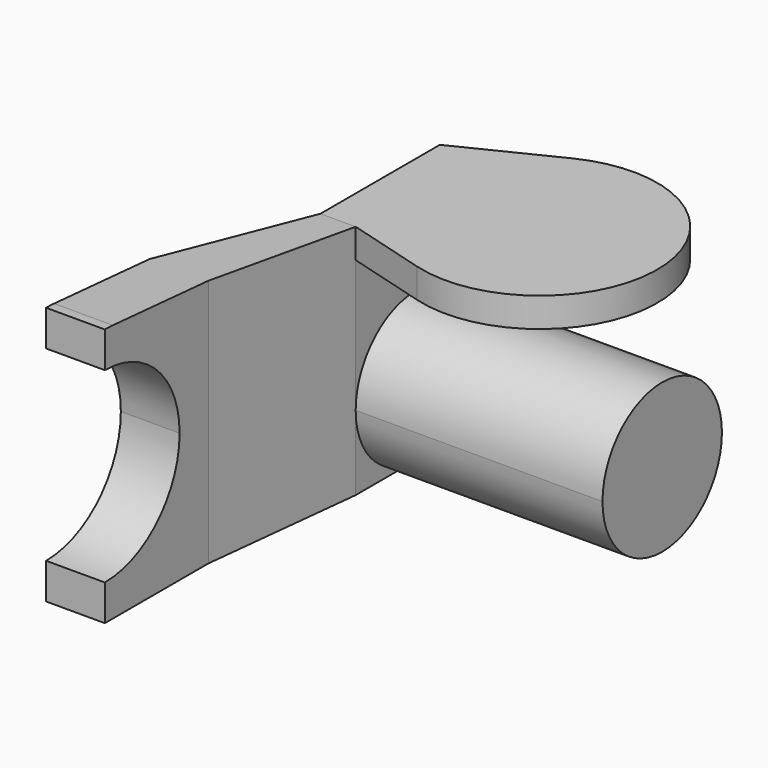
from build123d import *

# Parameters (mm, degrees)
F1_DEPTH      = 10
F2_DEPTH      = 3
F2_DEPTH_BACK = 3
F1_FACE_W     = 10
F1_FACE_H     = 42.3516603272
F2_FACE_W     = 6
F2_FACE_H     = 40.2
F5_DEPTH      = 5
F6_START      = 2
F6_DEPTH      = 43
F8_DEPTH      = 5


# Not quite as in the source:
# - a feature names something its author has since deleted; it is built from what else it names


with BuildPart() as f1:
    # F0 (on Right) → F1 (new body)
    with BuildSketch(Plane.YZ):
        with BuildLine():
            ThreePointArc((15.9, 0), (11.2429978209, -11.2429978209), (0, -15.9))
            Line((0, -15.9), (0, -22))
            ThreePointArc((0, -22), (15.5563491861, -15.5563491861), (22, 0))
            ThreePointArc((22, 0), (16.1495801051, 14.9395803966), (1.7099034157, 21.9334500321))
            ThreePointArc((1.7099034157, 21.9334500321), (0.8555989991, 21.9833562122), (0, 22))
            Line((0, 22), (0, 15.9))
            ThreePointArc((0, 15.9), (11.2429978209, 11.2429978209), (15.9, 0))
        make_face()
        with BuildLine():
            ThreePointArc((1.7099034157, 21.9334500321), (16.1495801051, 14.9395803966), (22, 0))
            Line((22, 0), (22, 20.3516603272))
            Line((22, 20.3516603272), (1.7099034157, 21.9334500321))
        make_face()
        with BuildLine():
            ThreePointArc((22, 0), (15.5563491861, -15.5563491861), (0, -22))
            Line((0, -22), (22, -22))
            Line((22, -22), (22, 0))
        make_face()
    extrude(amount=-F1_DEPTH)


with BuildPart() as f2:
    # F0 (on Right) → F2 (new body, two sides)
    with BuildSketch(Plane.YZ) as f2_sk:
        with BuildLine():
            Line((75, 18.2), (49.6, 18.2))
            Line((49.6, 18.2), (49.6, 13.2))
            Line((49.6, 13.2), (49.6, -9.3))
            ThreePointArc((49.6, -9.3), (62.3, 3.4), (75, -9.3))
            Line((75, -9.3), (75, 0))
            Line((75, 0), (75, 18.2))
        make_face()
        with BuildLine():
            ThreePointArc((49.6, -9.3), (53.3197438789, -18.2802561211), (62.3, -22))
            ThreePointArc((62.3, -22), (71.2802561211, -18.2802561211), (75, -9.3))
            ThreePointArc((75, -9.3), (62.3, 3.4), (49.6, -9.3))
        make_face()
        with BuildLine():
            Line((49.6, -9.3), (49.6, -22))
            Line((49.6, -22), (62.3, -22))
            ThreePointArc((62.3, -22), (53.3197438789, -18.2802561211), (49.6, -9.3))
        make_face()
    extrude(amount=F2_DEPTH)
    extrude(f2_sk.sketch, amount=-F2_DEPTH_BACK)


with BuildPart() as f3:
    # F1_face (on face) → F3 section 0
    with BuildSketch(Plane(origin=(-5, 22, -0.8241698364), x_dir=(-1, 0, 0), z_dir=(0, 1, 0))):
        Rectangle(F1_FACE_W, F1_FACE_H)
    # F2_face (on face) → F3 section 1
    with BuildSketch(Plane(origin=(0, 49.6, -1.9), x_dir=(1, 0, 0), z_dir=(0, -1, 0))):
        Rectangle(F2_FACE_W, F2_FACE_H)
    loft()


with BuildPart() as f1_1:
    add(f1.part)

    # F4: union F2, F3
    add(f2.part)
    add(f3.part)

    # F5 (cut): a face of the model
    f5_faces = [f1_1.faces().sort_by_distance(p)[0] for p in [
        (0, 62.3, 18.2),
    ]]
    extrude(f5_faces, amount=-F5_DEPTH, mode=Mode.SUBTRACT)


with BuildPart() as f6:
    # F0 (on Right) → F6 (new body)
    with BuildSketch(Plane.YZ.offset(F6_START)):
        with BuildLine():
            ThreePointArc((49.6, -9.3), (53.3197438789, -18.2802561211), (62.3, -22))
            ThreePointArc((62.3, -22), (71.2802561211, -18.2802561211), (75, -9.3))
            ThreePointArc((75, -9.3), (62.3, 3.4), (49.6, -9.3))
        make_face()
    extrude(amount=F6_DEPTH)


with BuildPart() as f8:
    # F7 (on face) → F8 (new body)
    with BuildSketch(Plane.XY.offset(13.2)):
        with BuildLine():
            ThreePointArc((16.5427559466, 45.7589374685), (34.0593349512, 49.0446735999), (42, 65))
            ThreePointArc((42, 65), (32.5735853544, 81.9764334521), (13.1800707248, 82.9501768119))
            ThreePointArc((13.1800707248, 82.9501768119), (6.9089457299, 78.1247887989), (3, 71.2449979984))
            Line((3, 71.2449979984), (3, 58.7550020016))
            ThreePointArc((3, 58.7550020016), (8.1521257946, 50.5696022234), (16.5427559466, 45.7589374685))
        make_face()
        with BuildLine():
            Line((3, 49.6), (16.5427559466, 45.7589374685))
            ThreePointArc((16.5427559466, 45.7589374685), (8.1521257946, 50.5696022234), (3, 58.7550020016))
            Line((3, 58.7550020016), (3, 49.6))
        make_face()
        with BuildLine():
            ThreePointArc((3, 58.7550020016), (2, 65), (3, 71.2449979984))
            Line((3, 71.2449979984), (3, 75))
            Line((3, 75), (-3, 75))
            Line((-3, 75), (-3, 49.6))
            Line((-3, 49.6), (3, 49.6))
            Line((3, 49.6), (3, 58.7550020016))
        make_face()
        with BuildLine():
            ThreePointArc((3, 71.2449979984), (6.9089457299, 78.1247887989), (13.1800707248, 82.9501768119))
            Line((13.1800707248, 82.9501768119), (-3, 75))
            Line((-3, 75), (3, 75))
            Line((3, 75), (3, 71.2449979984))
        make_face()
        with BuildLine():
            Line((3, 58.7550020016), (3, 71.2449979984))
            ThreePointArc((3, 71.2449979984), (2, 65), (3, 58.7550020016))
        make_face()
    extrude(amount=F8_DEPTH)


solid = Compound([f1_1.part, f6.part, f8.part])
